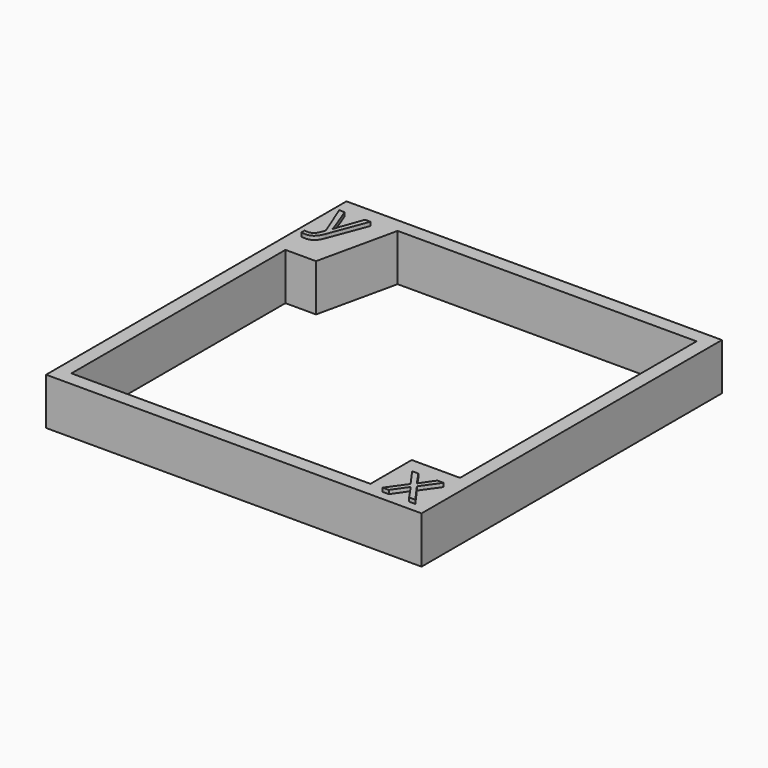
from build123d import *

# Parameters (mm, degrees)
F0_W           = 40
F0_H           = 40
F1_DEPTH       = 5
F2_TEXT_SIZE   = 6.6263759685
F2_TEXT_SIZE_2 = 7.1775371479
F3_DEPTH       = 0.4
F5_DEPTH       = 25


# Not quite as in the source:
# - Text() gives the source's letters only with a copy of the font that has no kerning and outlines rounded to 1/6400 em; it was checked with that copy


with BuildPart() as f1:
    # F0 (on Top) → F1 (new body)
    with BuildSketch(Plane.XY):
        Rectangle(F0_W, F0_H)
    extrude(amount=F1_DEPTH)

    # F2 (on face) → F3 (join)
    with BuildSketch(Plane.XY.offset(5)):
        with Locations((-19, 14.2290093027)):
            Text('y', F2_TEXT_SIZE, font='Open Sans', text_align=(TextAlign.LEFT, TextAlign.BOTTOM))
        with Locations((14.9177757471, -19)):
            Text('x', F2_TEXT_SIZE_2, font='Open Sans', text_align=(TextAlign.LEFT, TextAlign.BOTTOM))
    extrude(amount=F3_DEPTH)

    # F4 (on face) → F5 (cut)
    with BuildSketch(Plane.XY.offset(5)):
        Polygon((18.5, 18.5), (-13.349291145, 18.5), (-15.241282209, 10), (-18.5, 10), (-18.5, -18.5), (13.3537088093, -18.5), (13.3537088093, -13), (18.5, -13), align=None)
    extrude(amount=-F5_DEPTH, mode=Mode.SUBTRACT)


solid = f1.part
